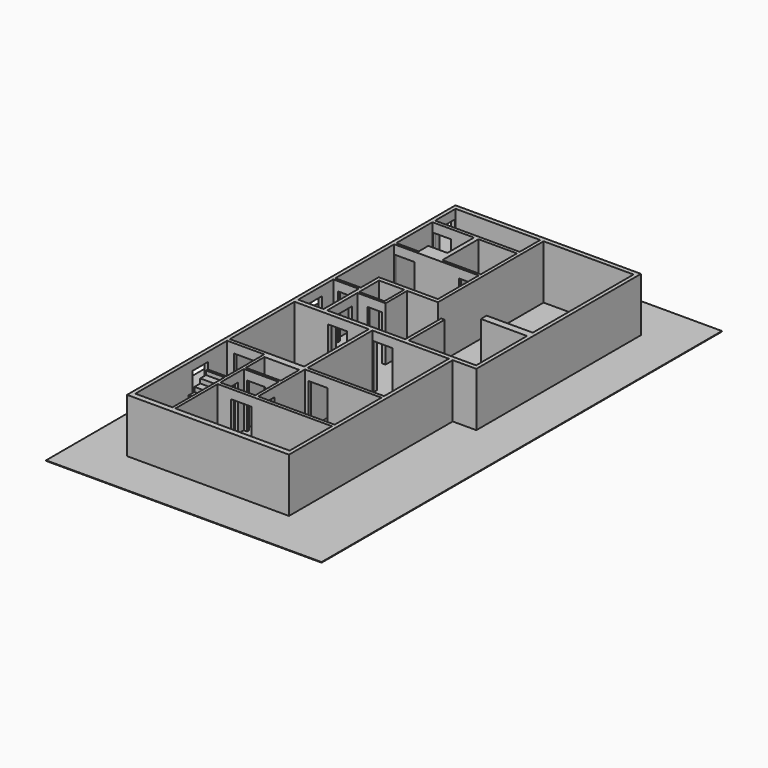
from build123d import *

# Parameters (mm, degrees)
F0_W     = 1650
F0_H     = 5100
F0_W_2   = 1550
F0_H_2   = 1300
F0_W_3   = 3300
F0_H_3   = 3600
F0_H_4   = 1035
F0_W_4   = 5080
F0_H_5   = 2350
F0_W_5   = 3400
F0_H_6   = 2600
F0_W_6   = 1130
F0_H_7   = 1950
F0_W_7   = 1120
F0_H_8   = 1100
F0_W_8   = 3760
F0_H_9   = 1140
F0_W_9   = 1710
F0_H_10  = 2010
F0_W_10  = 850
F0_H_11  = 530
F1_DEPTH = 2400
F3_START = -400
F2_W     = 170
F2_H     = 850
F2_W_2   = 800
F2_H_2   = 150
F2_W_3   = 880
F2_H_3   = 115
F2_W_4   = 870
F2_W_5   = 850
F2_H_4   = 880
F2_W_6   = 650
F2_H_5   = 100
F2_W_7   = 160
F2_H_6   = 200
F2_W_8   = 130
F2_W_9   = 900
F3_DEPTH = 2000
F4_W     = 12250
F4_H     = 22250
F5_DEPTH = 25
F7_START = 825
F7_DEPTH = 825
F8_DEPTH = 825


with BuildPart() as f1:
    # F0 (on Top) → F1 (new body)
    with BuildSketch(Plane.XY):
        Polygon((4125, 0), (-4125, 0), (-4125, -9150), (-4125, -18250), (3075, -18250), (3075, -9150), (4125, -9150), align=None)
        with Locations((-3130, -15450)):
            Rectangle(F0_W, F0_H, mode=Mode.SUBTRACT)
        with Locations((-1400, -14850)):
            Rectangle(F0_W_2, F0_H_2, mode=Mode.SUBTRACT)
        with Locations((-2305, -10950)):
            Rectangle(F0_W_3, F0_H_3, mode=Mode.SUBTRACT)
        with Locations((-1400, -13567.5)):
            Rectangle(F0_W_2, F0_H_4, mode=Mode.SUBTRACT)
        with Locations((365, -16825)):
            Rectangle(F0_W_4, F0_H_5, mode=Mode.SUBTRACT)
        with Locations((1205, -14200)):
            Rectangle(F0_W_5, F0_H_6, mode=Mode.SUBTRACT)
        with Locations((1205, -10950)):
            Rectangle(F0_W_5, F0_H_3, mode=Mode.SUBTRACT)
        with Locations((-3390, -7975)):
            Rectangle(F0_W_6, F0_H_7, mode=Mode.SUBTRACT)
        with Locations((-2105, -6620)):
            Rectangle(F0_W_7, F0_H_8, mode=Mode.SUBTRACT)
        Polygon((-3955, -5885), (-3955, -3615), (-195, -3615), (-195, -5885), (-2825, -5885), (-2825, -6885), (-3955, -6885), align=None, mode=Mode.SUBTRACT)
        Polygon((-3955, -3500), (-3955, -1490), (-2105, -1490), (-2105, -2970), (-2105, -3500), (-2955, -3500), align=None, mode=Mode.SUBTRACT)
        with Locations((-2075, -770)):
            Rectangle(F0_W_8, F0_H_9, mode=Mode.SUBTRACT)
        with Locations((-1050, -2495)):
            Rectangle(F0_W_9, F0_H_10, mode=Mode.SUBTRACT)
        Polygon((-45, -6070), (-45, -200), (3955, -200), (3955, -5800), (1905, -5800), (1905, -6120), (3955, -6120), (3955, -8950), (955, -8950), (955, -6950), (805, -6950), (805, -8950), (-2665, -8950), (-2665, -7270), (-1415, -7270), (-1415, -6070), align=None, mode=Mode.SUBTRACT)
        with Locations((-2530, -3235)):
            Rectangle(F0_W_10, F0_H_11)
    extrude(amount=F1_DEPTH)

    # F2 (on face) → F3 (cut)
    with BuildSketch(Plane.XY.offset(2400).offset(F3_START)):
        with Locations((-4040, -665)):
            Rectangle(F2_W, F2_H)
        with Locations((-3535, -1415)):
            Rectangle(F2_W_2, F2_H_2)
        with Locations((-3495, -3557.5)):
            Rectangle(F2_W_3, F2_H_3)
        with Locations((-640, -3557.5)):
            Rectangle(F2_W_4, F2_H_3)
        with Locations((-3330, -6942.5)):
            Rectangle(F2_W_5, F2_H_3)
        with Locations((-4040, -8060)):
            Rectangle(F2_W, F2_H_4)
        with Locations((-1890, -7220)):
            Rectangle(F2_W_6, F2_H_5)
        with Locations((-2745, -8010)):
            Rectangle(F2_W_7, F2_H_4)
        with Locations((-2040, -9050)):
            Rectangle(F2_W_5, F2_H_6)
        with Locations((-20, -9050)):
            Rectangle(F2_W_5, F2_H_6)
        with Locations((-3230, -12825)):
            Rectangle(F2_W_5, F2_H_2)
        with Locations((80, -12825)):
            Rectangle(F2_W_5, F2_H_2)
        with Locations((-1625, -14142.5)):
            Rectangle(F2_W_2, F2_H_3)
        with Locations((-560, -15040)):
            Rectangle(F2_W_8, F2_H_4)
        with Locations((-1125, -15575)):
            Rectangle(F2_W_9, F2_H_2)
        with Locations((-2240, -14960)):
            Rectangle(F2_W_8, F2_H_4)
        with Locations((-4040, -14390)):
            Rectangle(F2_W, F2_H_4)
    extrude(amount=-F3_DEPTH, mode=Mode.SUBTRACT)


with BuildPart() as f5:
    # F4 (on Top) → F5 (new body)
    with BuildSketch(Plane.XY):
        with Locations((0, -9125)):
            Rectangle(F4_W, F4_H)
    extrude(amount=-F5_DEPTH)


with BuildPart() as f7:
    # F6 (on face) → F7 (new body)
    with BuildSketch(Plane(origin=(-2305, 0, 0), x_dir=(0, -1, 0), z_dir=(-1, 0, 0)).offset(F7_START)):
        Polygon((16050, 220), (15730, 220), (15730, 0), (17680, 0), (17680, 820), (17010, 820), (16690, 820), (16690, 620), (16370, 620), (16370, 420), (16050, 420), align=None)
        Polygon((17010, 820), (17680, 820), (17680, 1020), (17010, 1020), (17010, 990), align=None)
    extrude(amount=F7_DEPTH)

    # F6 (on face) → F8 (join)
    with BuildSketch(Plane(origin=(-2305, 0, 0), x_dir=(0, -1, 0), z_dir=(-1, 0, 0))):
        Polygon((15400, 2000), (15400, 1734.2952563354), (16440.20652771, 1020), (17010, 990), (17010, 1020), (17010, 1220), (16690, 1220), (16690, 1420), (16370, 1420), (16370, 1620), (16068, 1620), (16068, 1820), (15748, 1820), (15748, 2020), (15428, 2020), (15428, 2220), (15108, 2220), (15108, 2400), (15008, 2400), (15008, 2003.4761670724), (15013.0622367264, 2000), align=None)
        Polygon((17010, 820), (17680, 820), (17680, 1020), (17010, 1020), (17010, 990), align=None)
    extrude(amount=F8_DEPTH)


solid = Compound([f1.part, f5.part, f7.part])
